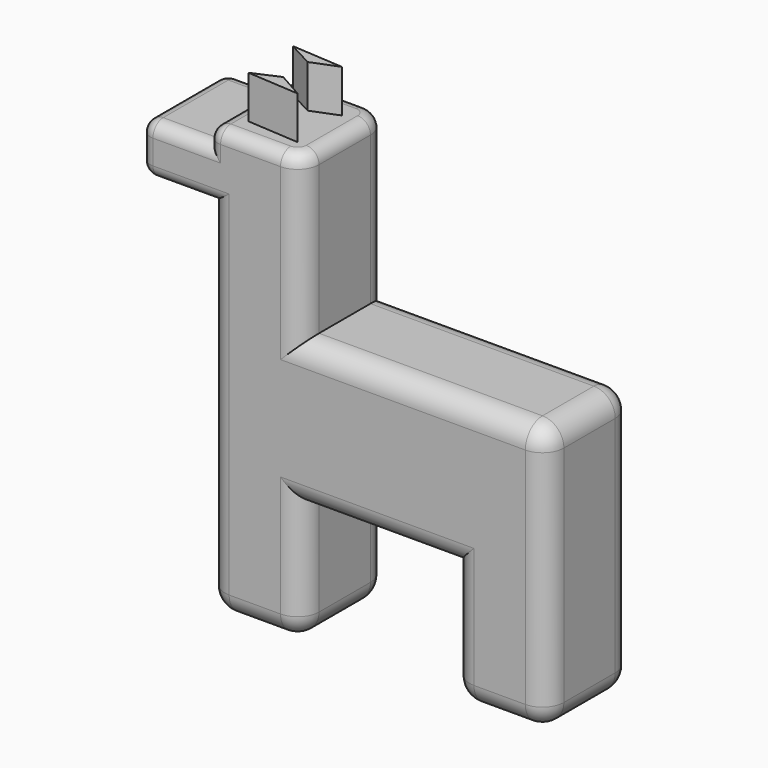
from build123d import *

# Parameters (mm, degrees)
F1_DEPTH      = 25
F2_R          = 3
F3_R          = 3
F4_T1_DEPTH   = 52.1931828042
F4_T3_DEPTH   = 15
F4_T5_DEPTH   = 52.3223032383
F4_T7_DEPTH   = 40.6846483105
F4_T9_DEPTH   = 79.471221308
F4_T11_DEPTH  = 23.1846483105
F4_T13_DEPTH  = 35.1931828042
F4_T15_DEPTH  = 12
F4_T17_DEPTH  = 29.5
F4_T19_DEPTH  = 37.6776967617
F4_T22_ANGLE  = 90
F4_T24_ANGLE  = 90
F4_S27_W      = 5.1
F4_S27_H      = 5.1
F4_T28_DEPTH  = 5.1
F4_S33_W      = 5.1
F4_S33_H      = 5.1
F4_T34_DEPTH  = 5.1
F4_S39_W      = 5.1
F4_S39_H      = 5.1
F4_T40_DEPTH  = 5.1
F4_S45_W      = 5.1
F4_S45_H      = 5.1
F4_T46_DEPTH  = 5.1
F4_S51_W      = 5.1
F4_S51_H      = 5.1
F4_T52_DEPTH  = 5.1
F4_S57_W      = 5.1
F4_S57_H      = 5.1
F4_T58_DEPTH  = 5.1
F4_S63_W      = 5.1
F4_S63_H      = 5.1
F4_T64_DEPTH  = 5.1
F4_S69_W      = 5.1
F4_S69_H      = 5.1
F4_T70_DEPTH  = 5.1
F4_T77_DEPTH  = 50.1776967617
F4_T81_DEPTH  = 64.6931828042
F4_T88_DEPTH  = 50.1776967617
F4_T92_DEPTH  = 64.6931828042
F4_T99_DEPTH  = 40.6846483105
F4_T103_DEPTH = 47.6931828042
F4_T110_DEPTH = 40.6846483105
F4_T114_DEPTH = 47.6931828042
F4_T121_DEPTH = 47.6931828042
F4_T125_DEPTH = 35.6846483105
F4_T132_DEPTH = 47.6931828042
F4_T136_DEPTH = 35.6846483105
F5_R          = 3
F6_T1_DEPTH   = 15
F6_S5_W       = 5
F6_S5_H       = 5
F6_T6_DEPTH   = 5
F6_S11_W      = 5
F6_S11_H      = 5
F6_T12_DEPTH  = 5
F8_DEPTH      = 10


# Not quite as in the source:
# - a fillet or chamfer that OpenCascade refuses, or shapes differently, is made with other operations: its cross-section is extruded or revolved along the edge and cut away or added


with BuildPart() as f1:
    # F0 (on Front) → F1 (new body)
    with BuildSketch(Plane.XZ):
        Polygon((-57.1931828042, 56.2865729975), (-57.1931828042, -28.1846483105), (-35.1931828042, -28.1846483105), (-35.1931828042, 0), (0, 0), (0, -28.1846483105), (22, -28.1846483105), (22, 0), (22, 34.1376549277), (-35.1931828042, 34.1376549277), (-35.1931828042, 71.8153516895), (-57.1931828042, 71.8153516895), (-57.1931828042, 67.9793483567), (-72.9995634697, 67.9793483567), (-72.9995634697, 56.2865729975), align=None)
    extrude(amount=F1_DEPTH)

    # F2
    f2_edges = [f1.edges().sort_by_distance(p)[0] for p in [
        (-46.193183, -25, 71.815352),
        (-35.193183, -12.5, 71.815352),
        (-46.193183, 0, 71.815352),
        (-65.096373, -25, 67.979348),
        (-65.096373, 0, 67.979348),
    ]]
    fillet(f2_edges, radius=F2_R)

    # F3
    f3_edges = [f1.edges().sort_by_distance(p)[0] for p in [
        (-57.193183, -12.5, 71.815352),
        (-72.999563, -12.5, 67.979348),
    ]]
    fillet(f3_edges, radius=F3_R)

    # F4: fillet of radius 5 on 22 edges, made by hand

    # F4_s2 → F4_t1 (cut)
    with BuildSketch(Plane.YZ.offset(-35.1931828042)):
        with BuildLine():
            ThreePointArc((-25, 29.1376549277), (-23.5355339059, 32.6731888337), (-20, 34.1376549277))
            Line((-20, 34.1376549277), (-25, 34.1376549277))
            Line((-25, 34.1376549277), (-25, 29.1376549277))
        make_face()
        with BuildLine():
            ThreePointArc((-5, 34.1376549277), (-1.4644660941, 32.6731888337), (0, 29.1376549277))
            Line((0, 29.1376549277), (0, 34.1376549277))
            Line((0, 34.1376549277), (-5, 34.1376549277))
        make_face()
    extrude(amount=F4_T1_DEPTH, mode=Mode.SUBTRACT)

    # F4_s4 → F4_t3 (cut)
    with BuildSketch(Plane.XZ.offset(5)):
        with BuildLine():
            ThreePointArc((17, 34.1376549277), (20.5355339059, 32.6731888337), (22, 29.1376549277))
            Line((22, 29.1376549277), (22, 34.1376549277))
            Line((22, 34.1376549277), (17, 34.1376549277))
        make_face()
        with BuildLine():
            ThreePointArc((-57.1931828042, -23.1846483105), (-55.7287167101, -26.7201822165), (-52.1931828042, -28.1846483105))
            Line((-52.1931828042, -28.1846483105), (-57.1931828042, -28.1846483105))
            Line((-57.1931828042, -28.1846483105), (-57.1931828042, -23.1846483105))
        make_face()
        with BuildLine():
            ThreePointArc((-35.1931828042, -23.1846483105), (-36.6576488983, -26.7201822165), (-40.1931828042, -28.1846483105))
            Line((-40.1931828042, -28.1846483105), (-35.1931828042, -28.1846483105))
            Line((-35.1931828042, -28.1846483105), (-35.1931828042, -23.1846483105))
        make_face()
        with BuildLine():
            ThreePointArc((22, -23.1846483105), (20.5355339059, -26.7201822165), (17, -28.1846483105))
            Line((17, -28.1846483105), (22, -28.1846483105))
            Line((22, -28.1846483105), (22, -23.1846483105))
        make_face()
    extrude(amount=F4_T3_DEPTH, mode=Mode.SUBTRACT)

    # F4_s6 → F4_t5 (cut)
    with BuildSketch(Plane.XY.offset(-23.1846483105)):
        with BuildLine():
            ThreePointArc((17, -25), (20.5355339059, -23.5355339059), (22, -20))
            Line((22, -20), (22, -25))
            Line((22, -25), (17, -25))
        make_face()
        with BuildLine():
            ThreePointArc((22, -5), (20.5355339059, -1.4644660941), (17, 0))
            Line((17, 0), (22, 0))
            Line((22, 0), (22, -5))
        make_face()
    extrude(amount=F4_T5_DEPTH, mode=Mode.SUBTRACT)

    # F4_s8 → F4_t7 (cut)
    with BuildSketch(Plane.XY.offset(-40.6846483105)):
        with BuildLine():
            ThreePointArc((0, -5), (1.4644660941, -1.4644660941), (5, 0))
            Line((5, 0), (0, 0))
            Line((0, 0), (0, -5))
        make_face()
        with BuildLine():
            ThreePointArc((5, -25), (1.4644660941, -23.5355339059), (0, -20))
            Line((0, -20), (0, -25))
            Line((0, -25), (5, -25))
        make_face()
    extrude(amount=F4_T7_DEPTH, mode=Mode.SUBTRACT)

    # F4_s10 → F4_t9 (cut)
    with BuildSketch(Plane.XY.offset(-23.1846483105)):
        with BuildLine():
            ThreePointArc((-57.1931828042, -5), (-55.7287167101, -1.4644660941), (-52.1931828042, 0))
            Line((-52.1931828042, 0), (-57.1931828042, 0))
            Line((-57.1931828042, 0), (-57.1931828042, -5))
        make_face()
        with BuildLine():
            ThreePointArc((-52.1931828042, -25), (-55.7287167101, -23.5355339059), (-57.1931828042, -20))
            Line((-57.1931828042, -20), (-57.1931828042, -25))
            Line((-57.1931828042, -25), (-52.1931828042, -25))
        make_face()
    extrude(amount=F4_T9_DEPTH, mode=Mode.SUBTRACT)

    # F4_s12 → F4_t11 (cut)
    with BuildSketch(Plane.XY.offset(-23.1846483105)):
        with BuildLine():
            ThreePointArc((-40.1931828042, -25), (-36.6576488983, -23.5355339059), (-35.1931828042, -20))
            Line((-35.1931828042, -20), (-35.1931828042, -25))
            Line((-35.1931828042, -25), (-40.1931828042, -25))
        make_face()
        with BuildLine():
            ThreePointArc((-35.1931828042, -5), (-36.6576488983, -1.4644660941), (-40.1931828042, 0))
            Line((-40.1931828042, 0), (-35.1931828042, 0))
            Line((-35.1931828042, 0), (-35.1931828042, -5))
        make_face()
    extrude(amount=F4_T11_DEPTH, mode=Mode.SUBTRACT)

    # F4_s14 → F4_t13 (cut)
    with BuildSketch(Plane.YZ.offset(-35.1931828042)):
        with BuildLine():
            ThreePointArc((-25, 5), (-23.5355339059, 1.4644660941), (-20, 0))
            Line((-20, 0), (-25, 0))
            Line((-25, 0), (-25, 5))
        make_face()
        with BuildLine():
            ThreePointArc((-5, 0), (-1.4644660941, 1.4644660941), (0, 5))
            Line((0, 5), (0, 0))
            Line((0, 0), (-5, 0))
        make_face()
    extrude(amount=F4_T13_DEPTH, mode=Mode.SUBTRACT)

    # F4_s16 → F4_t15 (cut)
    with BuildSketch(Plane.YZ.offset(-52.1931828042)):
        with BuildLine():
            ThreePointArc((-25, -23.1846483105), (-23.5355339059, -26.7201822165), (-20, -28.1846483105))
            Line((-20, -28.1846483105), (-25, -28.1846483105))
            Line((-25, -28.1846483105), (-25, -23.1846483105))
        make_face()
        with BuildLine():
            ThreePointArc((-5, -28.1846483105), (-1.4644660941, -26.7201822165), (0, -23.1846483105))
            Line((0, -23.1846483105), (0, -28.1846483105))
            Line((0, -28.1846483105), (-5, -28.1846483105))
        make_face()
    extrude(amount=F4_T15_DEPTH, mode=Mode.SUBTRACT)

    # F4_s18 → F4_t17 (cut)
    with BuildSketch(Plane.YZ.offset(-12.5)):
        with BuildLine():
            ThreePointArc((-25, -23.1846483105), (-23.5355339059, -26.7201822165), (-20, -28.1846483105))
            Line((-20, -28.1846483105), (-25, -28.1846483105))
            Line((-25, -28.1846483105), (-25, -23.1846483105))
        make_face()
        with BuildLine():
            ThreePointArc((-5, -28.1846483105), (-1.4644660941, -26.7201822165), (0, -23.1846483105))
            Line((0, -23.1846483105), (0, -28.1846483105))
            Line((0, -28.1846483105), (-5, -28.1846483105))
        make_face()
    extrude(amount=F4_T17_DEPTH, mode=Mode.SUBTRACT)

    # F4_s20 → F4_t19 (cut)
    with BuildSketch(Plane.XY.offset(34.1376549277)):
        with BuildLine():
            ThreePointArc((-40.1931828042, -25), (-36.6576488983, -23.5355339059), (-35.1931828042, -20))
            Line((-35.1931828042, -20), (-35.1931828042, -25))
            Line((-35.1931828042, -25), (-40.1931828042, -25))
        make_face()
        with BuildLine():
            ThreePointArc((-35.1931828042, -5), (-36.6576488983, -1.4644660941), (-40.1931828042, 0))
            Line((-40.1931828042, 0), (-35.1931828042, 0))
            Line((-35.1931828042, 0), (-35.1931828042, -5))
        make_face()
    extrude(amount=F4_T19_DEPTH, mode=Mode.SUBTRACT)

    # F4_s21 → F4_t22 (revolve, cut)
    with BuildSketch(Plane.XZ.offset(5)):
        with BuildLine():
            ThreePointArc((-38.1931828042, 71.8153516895), (-36.0718624607, 70.936672033), (-35.1931828042, 68.8153516895))
            Line((-35.1931828042, 68.8153516895), (-35.1931828042, 71.8153516895))
            Line((-35.1931828042, 71.8153516895), (-38.1931828042, 71.8153516895))
        make_face()
    revolve(axis=Axis((-40.1931828042, -5, 71.8153516895), (0, 0, 1)), revolution_arc=F4_T22_ANGLE, mode=Mode.SUBTRACT)

    # F4_s23 → F4_t24 (revolve, cut)
    with BuildSketch(Plane.YZ.offset(-40.1931828042)):
        with BuildLine():
            ThreePointArc((-22, 71.8153516895), (-24.1213203436, 70.936672033), (-25, 68.8153516895))
            Line((-25, 68.8153516895), (-25, 71.8153516895))
            Line((-25, 71.8153516895), (-22, 71.8153516895))
        make_face()
    revolve(axis=Axis((-40.1931828042, -20, 71.8153516895), (0, 0, 1)), revolution_arc=F4_T24_ANGLE, mode=Mode.SUBTRACT)


with BuildPart() as f4_tool26:
    # F4_s27 → F4_t28 (new body)
    with BuildSketch(Plane.XZ.offset(20)):
        with Locations((19.55, 31.6876549277)):
            Rectangle(F4_S27_W, F4_S27_H)
    extrude(amount=F4_T28_DEPTH)

    # F4_s29 → F4_t30 (revolve, cut)
    with BuildSketch(Plane(origin=(17, -20, 29.1376549277), x_dir=(-0.7071067812, 0, -0.7071067812), z_dir=(-0.7071067812, 0, 0.7071067812))):
        with BuildLine():
            ThreePointArc((0, -5), (5, 0), (0, 5))
            Line((0, 5), (0, -5))
        make_face()
    revolve(axis=Axis((17, -20, 29.1376549277), (0, -1, 0)), mode=Mode.SUBTRACT)


with BuildPart() as f1_1:
    add(f1.part)

    # F4_t25: cut F4_tool26
    add(f4_tool26.part, mode=Mode.SUBTRACT)


with BuildPart() as f4_tool32:
    # F4_s33 → F4_t34 (new body)
    with BuildSketch(Plane.XZ.offset(5)):
        with Locations((19.55, 31.6876549277)):
            Rectangle(F4_S33_W, F4_S33_H)
    extrude(amount=-F4_T34_DEPTH)

    # F4_s35 → F4_t36 (revolve, cut)
    with BuildSketch(Plane(origin=(17, -5, 29.1376549277), x_dir=(-0.7071067812, 0, -0.7071067812), z_dir=(0.7071067812, 0, -0.7071067812))):
        with BuildLine():
            ThreePointArc((0, -5), (5, 0), (0, 5))
            Line((0, 5), (0, -5))
        make_face()
    revolve(axis=Axis((17, -5, 29.1376549277), (0, 1, 0)), mode=Mode.SUBTRACT)


with BuildPart() as f1_2:
    add(f1_1.part)

    # F4_t31: cut F4_tool32
    add(f4_tool32.part, mode=Mode.SUBTRACT)


with BuildPart() as f4_tool38:
    # F4_s39 → F4_t40 (new body)
    with BuildSketch(Plane.XZ.offset(20)):
        with Locations((19.55, -25.7346483105)):
            Rectangle(F4_S39_W, F4_S39_H)
    extrude(amount=F4_T40_DEPTH)

    # F4_s41 → F4_t42 (revolve, cut)
    with BuildSketch(Plane(origin=(17, -20, -23.1846483105), x_dir=(-0.7071067812, 0, 0.7071067812), z_dir=(0.7071067812, 0, 0.7071067812))):
        with BuildLine():
            ThreePointArc((0, -5), (5, 0), (0, 5))
            Line((0, 5), (0, -5))
        make_face()
    revolve(axis=Axis((17, -20, -23.1846483105), (0, -1, 0)), mode=Mode.SUBTRACT)


with BuildPart() as f1_3:
    add(f1_2.part)

    # F4_t37: cut F4_tool38
    add(f4_tool38.part, mode=Mode.SUBTRACT)


with BuildPart() as f4_tool44:
    # F4_s45 → F4_t46 (new body)
    with BuildSketch(Plane.XZ.offset(5)):
        with Locations((-54.7431828042, -25.7346483105)):
            Rectangle(F4_S45_W, F4_S45_H)
    extrude(amount=-F4_T46_DEPTH)

    # F4_s47 → F4_t48 (revolve, cut)
    with BuildSketch(Plane(origin=(-52.1931828042, -5, -23.1846483105), x_dir=(0.7071067812, 0, 0.7071067812), z_dir=(-0.7071067812, 0, 0.7071067812))):
        with BuildLine():
            ThreePointArc((0, -5), (5, 0), (0, 5))
            Line((0, 5), (0, -5))
        make_face()
    revolve(axis=Axis((-52.1931828042, -5, -23.1846483105), (0, 1, 0)), mode=Mode.SUBTRACT)


with BuildPart() as f1_4:
    add(f1_3.part)

    # F4_t43: cut F4_tool44
    add(f4_tool44.part, mode=Mode.SUBTRACT)


with BuildPart() as f4_tool50:
    # F4_s51 → F4_t52 (new body)
    with BuildSketch(Plane.XZ.offset(20)):
        with Locations((-54.7431828042, -25.7346483105)):
            Rectangle(F4_S51_W, F4_S51_H)
    extrude(amount=F4_T52_DEPTH)

    # F4_s53 → F4_t54 (revolve, cut)
    with BuildSketch(Plane(origin=(-52.1931828042, -20, -23.1846483105), x_dir=(0.7071067812, 0, 0.7071067812), z_dir=(0.7071067812, 0, -0.7071067812))):
        with BuildLine():
            ThreePointArc((0, -5), (5, 0), (0, 5))
            Line((0, 5), (0, -5))
        make_face()
    revolve(axis=Axis((-52.1931828042, -20, -23.1846483105), (0, -1, 0)), mode=Mode.SUBTRACT)


with BuildPart() as f1_5:
    add(f1_4.part)

    # F4_t49: cut F4_tool50
    add(f4_tool50.part, mode=Mode.SUBTRACT)


with BuildPart() as f4_tool56:
    # F4_s57 → F4_t58 (new body)
    with BuildSketch(Plane.XZ.offset(20)):
        with Locations((-37.6431828042, -25.7346483105)):
            Rectangle(F4_S57_W, F4_S57_H)
    extrude(amount=F4_T58_DEPTH)

    # F4_s59 → F4_t60 (revolve, cut)
    with BuildSketch(Plane(origin=(-40.1931828042, -20, -23.1846483105), x_dir=(-0.7071067812, 0, 0.7071067812), z_dir=(0.7071067812, 0, 0.7071067812))):
        with BuildLine():
            ThreePointArc((0, -5), (5, 0), (0, 5))
            Line((0, 5), (0, -5))
        make_face()
    revolve(axis=Axis((-40.1931828042, -20, -23.1846483105), (0, -1, 0)), mode=Mode.SUBTRACT)


with BuildPart() as f1_6:
    add(f1_5.part)

    # F4_t55: cut F4_tool56
    add(f4_tool56.part, mode=Mode.SUBTRACT)


with BuildPart() as f4_tool62:
    # F4_s63 → F4_t64 (new body)
    with BuildSketch(Plane.XZ.offset(5)):
        with Locations((-37.6431828042, -25.7346483105)):
            Rectangle(F4_S63_W, F4_S63_H)
    extrude(amount=-F4_T64_DEPTH)

    # F4_s65 → F4_t66 (revolve, cut)
    with BuildSketch(Plane(origin=(-40.1931828042, -5, -23.1846483105), x_dir=(-0.7071067812, 0, 0.7071067812), z_dir=(-0.7071067812, 0, -0.7071067812))):
        with BuildLine():
            ThreePointArc((0, -5), (5, 0), (0, 5))
            Line((0, 5), (0, -5))
        make_face()
    revolve(axis=Axis((-40.1931828042, -5, -23.1846483105), (0, 1, 0)), mode=Mode.SUBTRACT)


with BuildPart() as f1_7:
    add(f1_6.part)

    # F4_t61: cut F4_tool62
    add(f4_tool62.part, mode=Mode.SUBTRACT)


with BuildPart() as f4_tool68:
    # F4_s69 → F4_t70 (new body)
    with BuildSketch(Plane.XY.offset(-23.1846483105)):
        with Locations((19.55, -2.45)):
            Rectangle(F4_S69_W, F4_S69_H)
    extrude(amount=-F4_T70_DEPTH)

    # F4_s71 → F4_t72 (revolve, cut)
    with BuildSketch(Plane(origin=(17, -5, -23.1846483105), x_dir=(-0.7071067812, -0.7071067812, 0), z_dir=(0.7071067812, -0.7071067812, 0))):
        with BuildLine():
            ThreePointArc((0, -5), (5, 0), (0, 5))
            Line((0, 5), (0, -5))
        make_face()
    revolve(axis=Axis((17, -5, -23.1846483105), (0, 0, -1)), mode=Mode.SUBTRACT)


with BuildPart() as f1_8:
    add(f1_7.part)

    # F4_t67: cut F4_tool68
    add(f4_tool68.part, mode=Mode.SUBTRACT)


with BuildPart() as f4_tool75:
    # F4_s76 → F4_t77 (new body)
    with BuildSketch(Plane.XY.offset(21.6376549277)):
        with BuildLine():
            ThreePointArc((-40.1931828042, -25), (-36.6576488983, -23.5355339059), (-35.1931828042, -20))
            Line((-35.1931828042, -20), (-35.1931828042, -25))
            Line((-35.1931828042, -25), (-40.1931828042, -25))
        make_face()
    extrude(amount=F4_T77_DEPTH)

    split(bisect_by=Plane.XY.offset(34.1376549277), keep=Keep.BOTTOM)


with BuildPart() as f4_tool79:
    # F4_s80 → F4_t81 (new body)
    with BuildSketch(Plane.YZ.offset(17)):
        with BuildLine():
            ThreePointArc((-25, 29.1376549277), (-23.5355339059, 32.6731888337), (-20, 34.1376549277))
            Line((-20, 34.1376549277), (-25, 34.1376549277))
            Line((-25, 34.1376549277), (-25, 29.1376549277))
        make_face()
    extrude(amount=-F4_T81_DEPTH)

    split(bisect_by=Plane.YZ.offset(-35.1931828042), keep=Keep.BOTTOM)


with BuildPart() as f4_tool75_1:
    add(f4_tool75.part)

    # F4_t83: intersect F4_tool79
    add(f4_tool79.part, mode=Mode.INTERSECT)


with BuildPart() as f1_9:
    add(f1_8.part)

    # F4_t73: cut F4_tool75
    add(f4_tool75_1.part, mode=Mode.SUBTRACT)


with BuildPart() as f4_tool86:
    # F4_s87 → F4_t88 (new body)
    with BuildSketch(Plane.XY.offset(21.6376549277)):
        with BuildLine():
            ThreePointArc((-35.1931828042, -5), (-36.6576488983, -1.4644660941), (-40.1931828042, 0))
            Line((-40.1931828042, 0), (-35.1931828042, 0))
            Line((-35.1931828042, 0), (-35.1931828042, -5))
        make_face()
    extrude(amount=F4_T88_DEPTH)

    split(bisect_by=Plane.XY.offset(34.1376549277), keep=Keep.BOTTOM)


with BuildPart() as f4_tool90:
    # F4_s91 → F4_t92 (new body)
    with BuildSketch(Plane.YZ.offset(17)):
        with BuildLine():
            ThreePointArc((-5, 34.1376549277), (-1.4644660941, 32.6731888337), (0, 29.1376549277))
            Line((0, 29.1376549277), (0, 34.1376549277))
            Line((0, 34.1376549277), (-5, 34.1376549277))
        make_face()
    extrude(amount=-F4_T92_DEPTH)

    split(bisect_by=Plane.YZ.offset(-35.1931828042), keep=Keep.BOTTOM)


with BuildPart() as f4_tool86_1:
    add(f4_tool86.part)

    # F4_t94: intersect F4_tool90
    add(f4_tool90.part, mode=Mode.INTERSECT)


with BuildPart() as f1_10:
    add(f1_9.part)

    # F4_t84: cut F4_tool86
    add(f4_tool86_1.part, mode=Mode.SUBTRACT)


with BuildPart() as f4_tool97:
    # F4_s98 → F4_t99 (new body)
    with BuildSketch(Plane.XY.offset(12.5)):
        with BuildLine():
            ThreePointArc((0, -5), (1.4644660941, -1.4644660941), (5, 0))
            Line((5, 0), (0, 0))
            Line((0, 0), (0, -5))
        make_face()
    extrude(amount=-F4_T99_DEPTH)

    split(bisect_by=Plane.XY, keep=Keep.TOP)


with BuildPart() as f4_tool101:
    # F4_s102 → F4_t103 (new body)
    with BuildSketch(Plane.YZ.offset(-35.1931828042)):
        with BuildLine():
            ThreePointArc((-5, 0), (-1.4644660941, 1.4644660941), (0, 5))
            Line((0, 5), (0, 0))
            Line((0, 0), (-5, 0))
        make_face()
    extrude(amount=F4_T103_DEPTH)

    split(bisect_by=Plane.YZ, keep=Keep.TOP)


with BuildPart() as f4_tool97_1:
    add(f4_tool97.part)

    # F4_t105: intersect F4_tool101
    add(f4_tool101.part, mode=Mode.INTERSECT)


with BuildPart() as f1_11:
    add(f1_10.part)

    # F4_t95: cut F4_tool97
    add(f4_tool97_1.part, mode=Mode.SUBTRACT)


with BuildPart() as f4_tool108:
    # F4_s109 → F4_t110 (new body)
    with BuildSketch(Plane.XY.offset(12.5)):
        with BuildLine():
            ThreePointArc((5, -25), (1.4644660941, -23.5355339059), (0, -20))
            Line((0, -20), (0, -25))
            Line((0, -25), (5, -25))
        make_face()
    extrude(amount=-F4_T110_DEPTH)

    split(bisect_by=Plane.XY, keep=Keep.TOP)


with BuildPart() as f4_tool112:
    # F4_s113 → F4_t114 (new body)
    with BuildSketch(Plane.YZ.offset(-35.1931828042)):
        with BuildLine():
            ThreePointArc((-25, 5), (-23.5355339059, 1.4644660941), (-20, 0))
            Line((-20, 0), (-25, 0))
            Line((-25, 0), (-25, 5))
        make_face()
    extrude(amount=F4_T114_DEPTH)

    split(bisect_by=Plane.YZ, keep=Keep.TOP)


with BuildPart() as f4_tool108_1:
    add(f4_tool108.part)

    # F4_t116: intersect F4_tool112
    add(f4_tool112.part, mode=Mode.INTERSECT)


with BuildPart() as f1_12:
    add(f1_11.part)

    # F4_t106: cut F4_tool108
    add(f4_tool108_1.part, mode=Mode.SUBTRACT)


with BuildPart() as f4_tool119:
    # F4_s120 → F4_t121 (new body)
    with BuildSketch(Plane.YZ.offset(-47.6931828042)):
        with BuildLine():
            ThreePointArc((-25, 5), (-23.5355339059, 1.4644660941), (-20, 0))
            Line((-20, 0), (-25, 0))
            Line((-25, 0), (-25, 5))
        make_face()
    extrude(amount=F4_T121_DEPTH)

    split(bisect_by=Plane.YZ.offset(-35.1931828042), keep=Keep.BOTTOM)


with BuildPart() as f4_tool123:
    # F4_s124 → F4_t125 (new body)
    with BuildSketch(Plane.XY.offset(-23.1846483105)):
        with BuildLine():
            ThreePointArc((-40.1931828042, -25), (-36.6576488983, -23.5355339059), (-35.1931828042, -20))
            Line((-35.1931828042, -20), (-35.1931828042, -25))
            Line((-35.1931828042, -25), (-40.1931828042, -25))
        make_face()
    extrude(amount=F4_T125_DEPTH)

    split(bisect_by=Plane.XY, keep=Keep.TOP)


with BuildPart() as f4_tool119_1:
    add(f4_tool119.part)

    # F4_t127: intersect F4_tool123
    add(f4_tool123.part, mode=Mode.INTERSECT)


with BuildPart() as f1_13:
    add(f1_12.part)

    # F4_t117: cut F4_tool119
    add(f4_tool119_1.part, mode=Mode.SUBTRACT)


with BuildPart() as f4_tool130:
    # F4_s131 → F4_t132 (new body)
    with BuildSketch(Plane.YZ.offset(-47.6931828042)):
        with BuildLine():
            ThreePointArc((-5, 0), (-1.4644660941, 1.4644660941), (0, 5))
            Line((0, 5), (0, 0))
            Line((0, 0), (-5, 0))
        make_face()
    extrude(amount=F4_T132_DEPTH)

    split(bisect_by=Plane.YZ.offset(-35.1931828042), keep=Keep.BOTTOM)


with BuildPart() as f4_tool134:
    # F4_s135 → F4_t136 (new body)
    with BuildSketch(Plane.XY.offset(-23.1846483105)):
        with BuildLine():
            ThreePointArc((-35.1931828042, -5), (-36.6576488983, -1.4644660941), (-40.1931828042, 0))
            Line((-40.1931828042, 0), (-35.1931828042, 0))
            Line((-35.1931828042, 0), (-35.1931828042, -5))
        make_face()
    extrude(amount=F4_T136_DEPTH)

    split(bisect_by=Plane.XY, keep=Keep.TOP)


with BuildPart() as f4_tool130_1:
    add(f4_tool130.part)

    # F4_t138: intersect F4_tool134
    add(f4_tool134.part, mode=Mode.INTERSECT)


with BuildPart() as f1_14:
    add(f1_13.part)

    # F4_t128: cut F4_tool130
    add(f4_tool130_1.part, mode=Mode.SUBTRACT)

    # F5
    f5_edges = [f1_14.edges().sort_by_distance(p)[0] for p in [
        (-72.999563, -12.5, 56.286573),
        (-61.096373, -25, 56.286573),
        (-61.096373, 0, 56.286573),
        (-72.120884, -0.87868, 56.286573),
        (-72.120884, -24.12132, 56.286573),
    ]]
    fillet(f5_edges, radius=F5_R)

    # F6: fillet of radius 5 on 1 edges, made by hand

    # F6_s2 → F6_t1 (cut)
    with BuildSketch(Plane.XZ.offset(5)):
        with BuildLine():
            ThreePointArc((0, -23.1846483105), (1.4644660941, -26.7201822165), (5, -28.1846483105))
            Line((5, -28.1846483105), (0, -28.1846483105))
            Line((0, -28.1846483105), (0, -23.1846483105))
        make_face()
    extrude(amount=F6_T1_DEPTH, mode=Mode.SUBTRACT)


with BuildPart() as f6_tool4:
    # F6_s5 → F6_t6 (new body)
    with BuildSketch(Plane.YZ.offset(5)):
        with Locations((-2.5, -25.6846483105)):
            Rectangle(F6_S5_W, F6_S5_H)
    extrude(amount=-F6_T6_DEPTH)

    # F6_s7 → F6_t8 (revolve, cut)
    with BuildSketch(Plane(origin=(5, -5, -23.1846483105), x_dir=(0, -0.7071067812, 0.7071067812), z_dir=(0, -0.7071067812, -0.7071067812))):
        with BuildLine():
            ThreePointArc((0, -5), (5, 0), (0, 5))
            Line((0, 5), (0, -5))
        make_face()
    revolve(axis=Axis((5, -5, -23.1846483105), (-1, 0, 0)), mode=Mode.SUBTRACT)


with BuildPart() as f1_15:
    add(f1_14.part)

    # F6_t3: cut F6_tool4
    add(f6_tool4.part, mode=Mode.SUBTRACT)


with BuildPart() as f6_tool10:
    # F6_s11 → F6_t12 (new body)
    with BuildSketch(Plane.YZ.offset(5)):
        with Locations((-22.5, -25.6846483105)):
            Rectangle(F6_S11_W, F6_S11_H)
    extrude(amount=-F6_T12_DEPTH)

    # F6_s13 → F6_t14 (revolve, cut)
    with BuildSketch(Plane(origin=(5, -20, -23.1846483105), x_dir=(0, 0.7071067812, 0.7071067812), z_dir=(0, -0.7071067812, 0.7071067812))):
        with BuildLine():
            ThreePointArc((0, -5), (5, 0), (0, 5))
            Line((0, 5), (0, -5))
        make_face()
    revolve(axis=Axis((5, -20, -23.1846483105), (-1, 0, 0)), mode=Mode.SUBTRACT)


with BuildPart() as f1_16:
    add(f1_15.part)

    # F6_t9: cut F6_tool10
    add(f6_tool10.part, mode=Mode.SUBTRACT)

    # F7 (on face) → F8 (join)
    with BuildSketch(Plane.XY.offset(71.8153516895)):
        Polygon((-46.3257431984, -16.549365595), (-52.3090921342, -19.1820412874), (-40.1931828042, -20), align=None)
        Polygon((-40.4822512322, -6.7235301125), (-52.5981605622, -5.9055713999), (-46.5402058972, -9.130010847), align=None)
    extrude(amount=F8_DEPTH)


solid = f1_16.part
